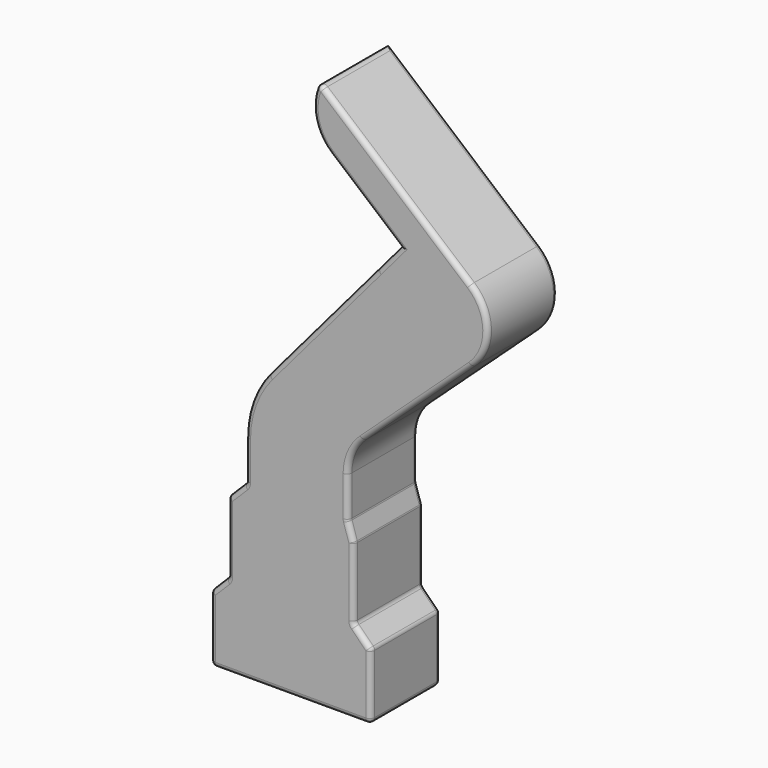
from build123d import *

# Parameters (mm, degrees)
F1_DEPTH    = 90
F2_T1_DEPTH = 507.1106760185
F2_T3_DEPTH = 372.5735965904
F3_R        = 5
F4_DEPTH    = 70
F5_W        = 86.5122303367
F5_H        = 49.2804106325
F6_DEPTH    = 170


# Not quite as in the source:
# - a fillet or chamfer that OpenCascade refuses, or shapes differently, is made with other operations: its cross-section is extruded or revolved along the edge and cut away or added


with BuildPart() as f1:
    # F0 (on Front) → F1 (new body)
    with BuildSketch(Plane.XZ):
        with BuildLine():
            Line((-126.2623920763, -193.7024648741), (-126.2623920763, -261.8315013925))
            Line((-126.2623920763, -261.8315013925), (39.092946983, -261.8315013925))
            Line((39.092946983, -261.8315013925), (39.092946983, -193.7024648741))
            Line((39.092946983, -193.7024648741), (21.4152774533, -176.0247953445))
            Line((21.4152774533, -176.0247953445), (21.4152774533, -102.6550637093))
            Line((21.4152774533, -102.6550637093), (15.5539703198, -84.1264084333))
            Line((15.5539703198, -84.1264084333), (15.5539703198, -42.2008474989))
            ThreePointArc((15.5539703198, -42.2008474989), (19.6898884351, -22.4740848198), (31.401046165, -6.0698241209))
            Line((31.401046165, -6.0698241209), (185.2309488965, 135.5598457642))
            Line((185.2309488965, 135.5598457642), (-14.4236341973, 305.266241394))
            Line((-14.4236341973, 305.266241394), (-66.2712781132, 297.6301199255))
            Line((-66.2712781132, 297.6301199255), (-11.4975965547, 251.0724906007))
            Line((-11.4975965547, 251.0724906007), (69.4938383905, 182.2297708973))
            Line((69.4938383905, 182.2297708973), (46.0270096541, 154.6217370896))
            Line((46.0270096541, 154.6217370896), (-66.2712781132, 22.5061044222))
            ThreePointArc((-66.2712781132, 22.5061044222), (-83.9215394862, -7.7309119674), (-90.0560672706, -42.2008474989))
            Line((-90.0560672706, -42.2008474989), (-90.0560672706, -84.1264084333))
            Line((-90.0560672706, -84.1264084333), (-108.5847225467, -102.6550637093))
            Line((-108.5847225467, -102.6550637093), (-108.5847225467, -176.0247953445))
            Line((-108.5847225467, -176.0247953445), (-126.2623920763, -193.7024648741))
        make_face()
    extrude(amount=F1_DEPTH)

    # F2: fillet of radius 50 on 2 edges, made by hand

    # F2_s2 → F2_t1 (cut)
    with BuildSketch(Plane.XZ.offset(-208.5553380092)):
        with BuildLine():
            ThreePointArc((-14.4236341973, 305.266241394), (-19.4476593821, 272.3668104124), (-2.7086733301, 243.6019058598))
            Line((-2.7086733301, 243.6019058598), (-66.2712781132, 297.6301199255))
            Line((-66.2712781132, 297.6301199255), (-14.4236341973, 305.266241394))
        make_face()
    extrude(amount=F2_T1_DEPTH, mode=Mode.SUBTRACT)

    # F2_s4 → F2_t3 (cut)
    with BuildSketch(Plane.XZ.offset(-141.2867982952)):
        with BuildLine():
            ThreePointArc((142.1701622159, 172.1615144427), (159.7779231252, 135.0553624638), (143.6543137068, 97.2806489872))
            Line((143.6543137068, 97.2806489872), (185.2309488965, 135.5598457642))
            Line((185.2309488965, 135.5598457642), (142.1701622159, 172.1615144427))
        make_face()
    extrude(amount=F2_T3_DEPTH, mode=Mode.SUBTRACT)

    # F3
    f3_edges = [f1.edges().sort_by_distance(p)[0] for p in [
        (39.092947, -45, -193.702465),
        (21.415277, -45, -176.024795),
        (30.254112, 0, -184.86363),
        (30.254112, -90, -184.86363),
        (-108.584723, 0, -139.33993),
        (-108.584723, -45, -176.024795),
        (-126.262392, -45, -193.702465),
        (-117.423557, 0, -184.86363),
        (-117.423557, -90, -184.86363),
        (-126.262392, -45, -261.831501),
        (-126.262392, 0, -227.766983),
        (-126.262392, -90, -227.766983),
        (-108.584723, -45, -102.655064),
        (-90.056067, -45, -42.200847),
        (-90.056067, -45, -84.126408),
        (-90.056067, 0, -63.163628),
        (-90.056067, -90, -63.163628),
        (-66.271278, -45, 22.506104),
        (-83.921539, 0, -7.730912),
        (-83.921539, -90, -7.730912),
        (63.873264, 0, 238.713878),
        (-14.423634, -45, 305.266241),
        (63.873264, -90, 238.713878),
        (142.170162, -45, 172.161514),
        (39.092947, -45, -261.831501),
        (39.092947, 0, -227.766983),
        (39.092947, -90, -227.766983),
        (-43.584723, 0, -261.831501),
        (1.61128, -90, 102.367938),
        (33.392583, -90, 212.915838),
        (-19.447659, -90, 272.36681),
        (159.777923, -90, 135.055362),
        (87.52768, -90, 45.605412),
        (19.689888, -90, -22.474085),
        (15.55397, -90, -63.163628),
        (18.484624, -90, -93.390736),
        (21.415277, -90, -139.33993),
        (-43.584723, -90, -261.831501),
        (-108.584723, -90, -139.33993),
        (-99.320395, -90, -93.390736),
        (21.415277, -45, -102.655064),
        (15.55397, -45, -84.126408),
        (18.484624, 0, -93.390736),
        (1.61128, 0, 102.367938),
        (159.777923, 0, 135.055362),
        (87.52768, 0, 45.605412),
        (19.689888, 0, -22.474085),
        (15.55397, 0, -63.163628),
        (21.415277, 0, -139.33993),
        (-99.320395, 0, -93.390736),
    ]]
    fillet(f3_edges, radius=F3_R)

    # F4 (cut): a face of the model
    f4_faces = [f1.faces().sort_by_distance(p)[0] for p in [
        (-43.5847225467, -45, -261.8315013925),
    ]]
    extrude(f4_faces, amount=-F4_DEPTH, mode=Mode.SUBTRACT)

    # F5 (on face) → F6 (cut)
    with BuildSketch(Plane(origin=(0, 0, -191.8315013925), x_dir=(1, 0, 0), z_dir=(0, 0, -1))):
        with Locations((-43.2561151683, 43.8658641651)):
            Rectangle(F5_W, F5_H)
    extrude(amount=-F6_DEPTH, mode=Mode.SUBTRACT)


solid = f1.part
